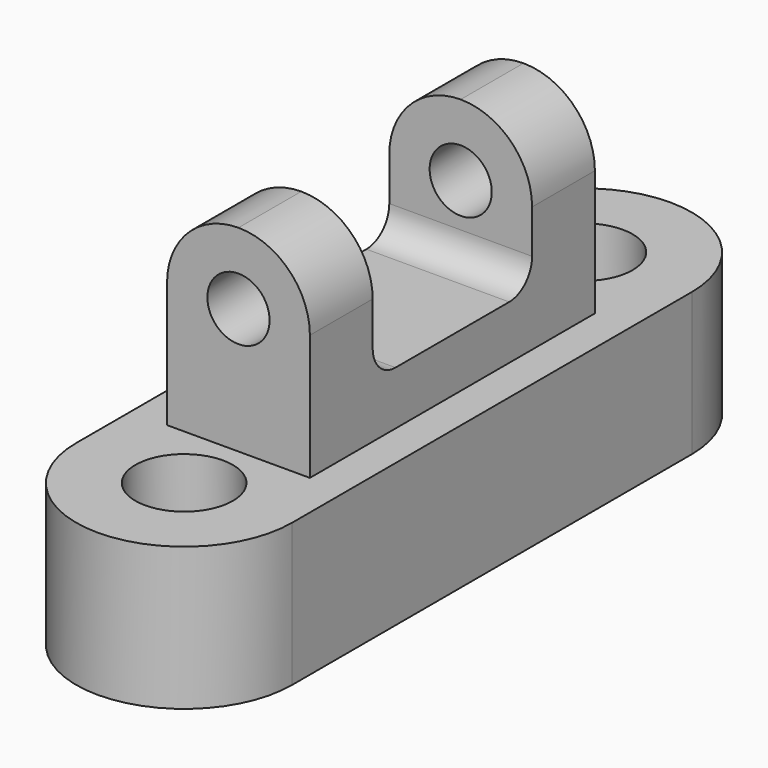
from build123d import *

# Parameters (mm, degrees)
F0_R      = 8.6637425689
F1_DEPTH  = 25.4
F3_DEPTH  = 12.7
F4_R      = 5.08
F5_R      = 5.08
F6_R      = 12.7
F7_R      = 12.69999
F8_R      = 12.7
F9_R      = 12.69999
F10_R     = 5.5257991494
F11_DEPTH = 25.4
F12_R     = 5.5331253453
F13_DEPTH = 25.4


# Not quite as in the source:
# - a fillet or chamfer is up to 0.001 mm smaller than in the source, because OpenCascade refuses the exact size


with BuildPart() as f1:
    # F0 (on Top) → F1 (new body)
    with BuildSketch(Plane.XY):
        with BuildLine():
            ThreePointArc((19.1970299929, 44.4350838661), (0, 63.6321138591), (-19.1970299929, 44.4350838661))
            Line((-19.1970299929, 44.4350838661), (-19.1970299929, -44.4350838661))
            ThreePointArc((-19.1970299929, -44.4350838661), (0, -63.6321138591), (19.1970299929, -44.4350838661))
            Line((19.1970299929, -44.4350838661), (19.1970299929, 44.4350838661))
        make_face()
        with Locations((0, -44.4350838661)):
            Circle(F0_R, mode=Mode.SUBTRACT)
        with Locations((0, 44.4350838661)):
            Circle(F0_R, mode=Mode.SUBTRACT)
    extrude(amount=-F1_DEPTH)

    # F2 (on Right) → F3 (join, symmetric)
    with BuildSketch(Plane.YZ):
        Polygon((-32.3530361056, 35.0379385054), (-32.3530361056, 0), (31.0105849057, 0), (31.0105849057, 35.0379385054), (17.0491095632, 35.0379385054), (17.0491095632, 9.5313927159), (-18.3915607631, 9.5313927159), (-18.3915607631, 35.0379385054), align=None)
    extrude(amount=F3_DEPTH, both=True)

    # F4
    f4_edges = [f1.edges().sort_by_distance(p)[0] for p in [
        (0, -18.391561, 9.531393),
    ]]
    fillet(f4_edges, radius=F4_R)

    # F5
    f5_edges = [f1.edges().sort_by_distance(p)[0] for p in [
        (0, 17.04911, 9.531393),
    ]]
    fillet(f5_edges, radius=F5_R)

    # F6
    f6_edges = [f1.edges().sort_by_distance(p)[0] for p in [
        (12.7, -25.372298, 35.037939),
    ]]
    fillet(f6_edges, radius=F6_R)

    # F7 (radius 12.7 in the source; OpenCascade refuses exactly that, so slightly less here)
    f7_edges = [f1.edges().sort_by_distance(p)[0] for p in [
        (-12.7, -25.372298, 35.037939),
    ]]
    fillet(f7_edges, radius=F7_R)

    # F8
    f8_edges = [f1.edges().sort_by_distance(p)[0] for p in [
        (12.7, 24.029847, 35.037939),
    ]]
    fillet(f8_edges, radius=F8_R)

    # F9 (radius 12.7 in the source; OpenCascade refuses exactly that, so slightly less here)
    f9_edges = [f1.edges().sort_by_distance(p)[0] for p in [
        (-12.7, 24.029847, 35.037939),
    ]]
    fillet(f9_edges, radius=F9_R)

    # F10 (on face) → F11 (cut)
    with BuildSketch(Plane(origin=(0, 31.0105849057, 0), x_dir=(-1, 0, 0), z_dir=(0, 1, 0))):
        with Locations((0, 22.3379385054)):
            Circle(F10_R)
    extrude(amount=-F11_DEPTH, mode=Mode.SUBTRACT)

    # F12 (on face) → F13 (cut)
    with BuildSketch(Plane.XZ.offset(32.3530361056)):
        with Locations((0, 22.3379385054)):
            Circle(F12_R)
    extrude(amount=-F13_DEPTH, mode=Mode.SUBTRACT)


solid = f1.part
